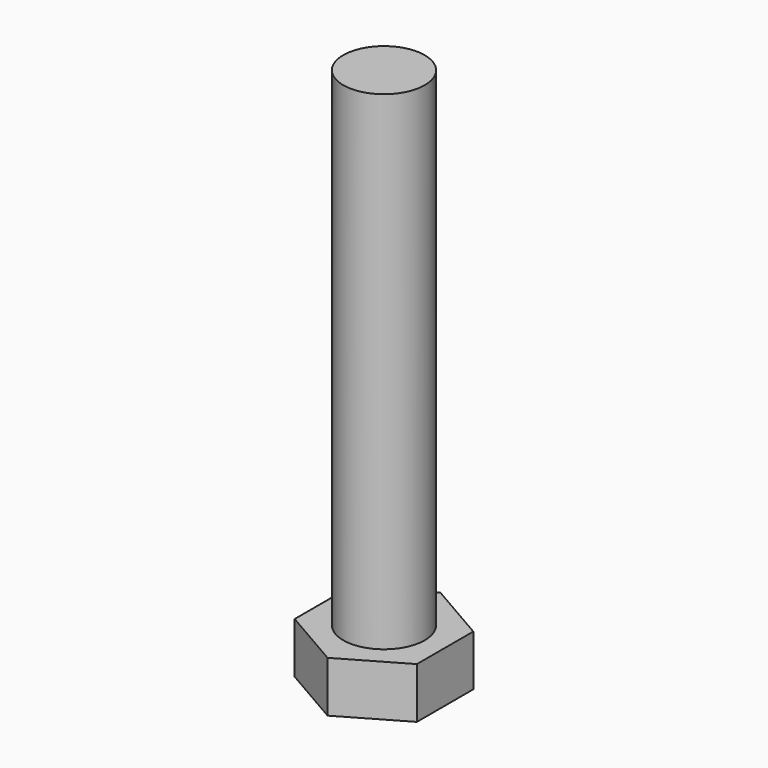
from build123d import *

# Parameters (mm, degrees)
F1_R     = 6.35
F2_DEPTH = 7.9375
F3_DEPTH = 84.1375


# Not quite as in the source:
# - a variable given as a bare number and used for a length is read in inches; the dataset says mm whatever the document's units were


with BuildPart() as f2:
    # F1 (on Top) → F2 (new body)
    with BuildSketch(Plane.XY):
        Polygon((9.525, -5.499261314), (9.525, 5.499261314), (0, 10.9985226281), (-9.525, 5.499261314), (-9.525, -5.499261314), (0, -10.9985226281), align=None)
        Circle(F1_R, mode=Mode.SUBTRACT)
    extrude(amount=F2_DEPTH)

    # F1 (on Top) → F3 (join)
    with BuildSketch(Plane.XY):
        Circle(F1_R)
    extrude(amount=F3_DEPTH)


solid = f2.part
